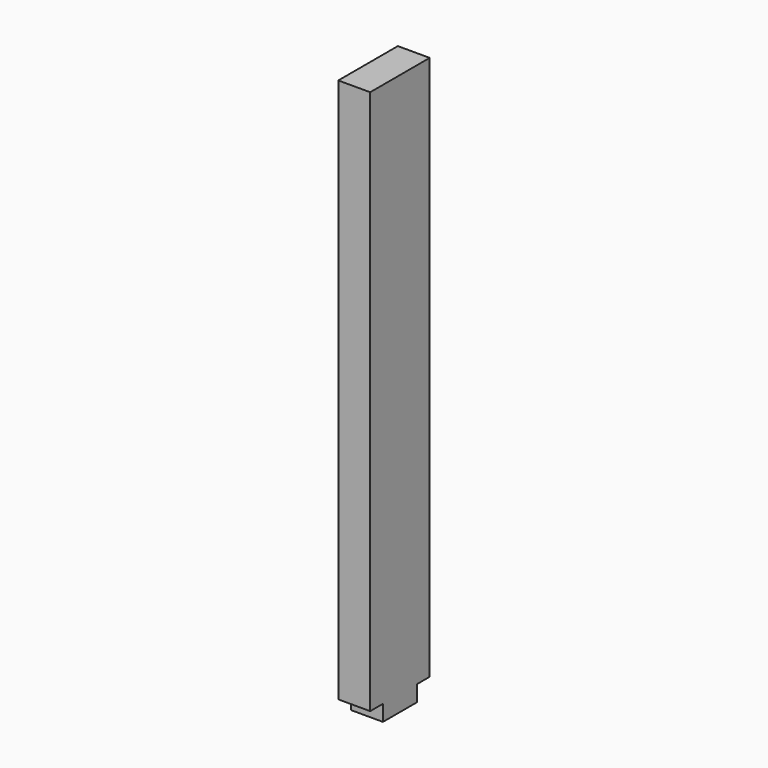
from build123d import *

# Parameters (mm, degrees)
F0_W     = 38.1
F0_H     = 88.9
F1_DEPTH = 650.95
F2_W     = 38.1
F2_H     = 50.8
F3_DEPTH = 19.05


# Not quite as in the source:
# - a length typed as a fraction of an inch, garbled in the dataset ("3 / 203.2 mm" for 3/8 in), is restored


with BuildPart() as f1:
    # F0 (on Top) → F1 (new body)
    with BuildSketch(Plane.XY):
        with Locations((19.05, 44.45)):
            Rectangle(F0_W, F0_H)
    extrude(amount=F1_DEPTH)

    # F2 (on face) → F3 (join)
    with BuildSketch(Plane(origin=(0, 0, 0), x_dir=(1, 0, 0), z_dir=(0, 0, -1))):
        with Locations((19.05, -44.45)):
            Rectangle(F2_W, F2_H)
    extrude(amount=F3_DEPTH)


solid = f1.part
